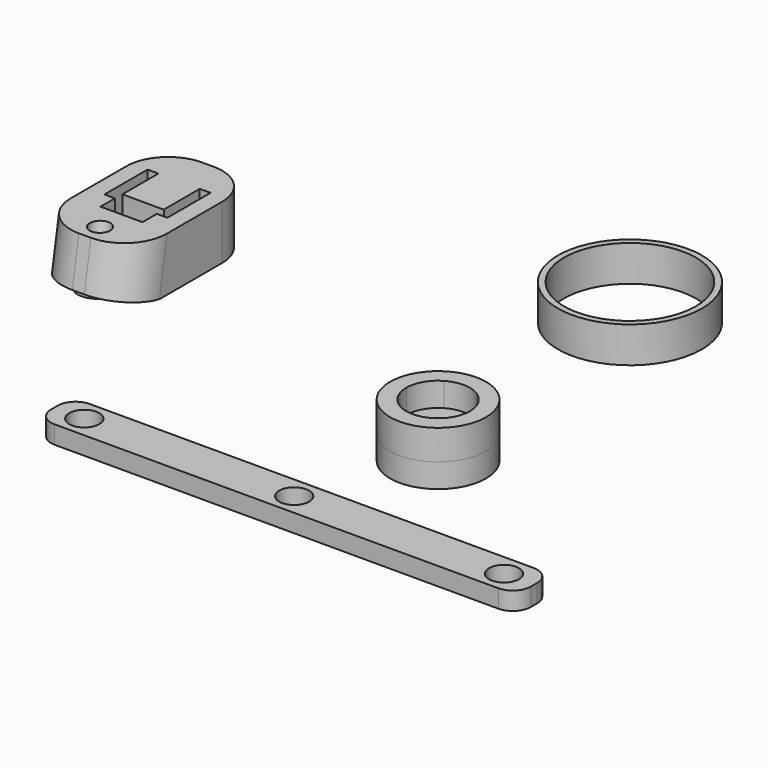
from build123d import *

# Parameters (mm, degrees)
F0_R         = 8
F1_DEPTH     = 4
F2_DEPTH     = 5
F0_R_2       = 2.5
F3_DEPTH     = 1
F4_DEPTH     = 3
F0_R_3       = 12
F0_R_4       = 11
F5_DEPTH     = 6
F0_W         = 16
F0_H         = 7
F0_H_2       = 20
F6_DEPTH     = 9
F8_W         = 16
F8_H         = 7.1079862832
F8_R         = 2.4
F8_R_2       = 1.7
F9_DEPTH     = 11.0033706387
F10_DEPTH    = 16.6784377721
F11_DEPTH    = 0.7
F12_R        = 2.3
F13_DEPTH    = 20
F8_H_2       = 1.3485015869
F14_DEPTH    = 16.6784377721
F15_T1_DEPTH = 44
F15_T3_DEPTH = 42.8855097467


# Not quite as in the source:
# - a fillet or chamfer that OpenCascade refuses, or shapes differently, is made with other operations: its cross-section is extruded or revolved along the edge and cut away or added


with BuildPart() as f1:
    # F0 (on Top) → F1 (new body)
    with BuildSketch(Plane.XY):
        Circle(F0_R)
        Polygon((5.3, 3.0599564267), (5.3, 0), (5.3, -3.0599564267), (2.6500008794, -4.5899341324), (0, -6.1199128534), (-2.6500009439, -4.5899340951), (-5.3, -3.0599564267), (-5.3, 0), (-5.3, 3.0599564267), (-2.6500008588, 4.5899341442), (0, 6.1199128534), (2.6500008831, 4.5899341302), align=None, mode=Mode.SUBTRACT)
    extrude(amount=-F1_DEPTH)

    # F0 (on Top) → F2 (join)
    with BuildSketch(Plane.XY):
        Circle(F0_R)
        Polygon((5.3, 3.0599564267), (5.3, 0), (5.3, -3.0599564267), (2.6500008794, -4.5899341324), (0, -6.1199128534), (-2.6500009439, -4.5899340951), (-5.3, -3.0599564267), (-5.3, 0), (-5.3, 3.0599564267), (-2.6500008588, 4.5899341442), (0, 6.1199128534), (2.6500008831, 4.5899341302), align=None, mode=Mode.SUBTRACT)
        with BuildLine():
            Line((0, -6.1199128534), (2.6500008794, -4.5899341324))
            ThreePointArc((2.6500008794, -4.5899341324), (-3.73e-08, -5.3), (-2.6500009439, -4.5899340951))
            Line((-2.6500009439, -4.5899340951), (0, -6.1199128534))
        make_face()
        with BuildLine():
            Line((-5.3, -3.0599564267), (-2.6500009439, -4.5899340951))
            ThreePointArc((-2.6500009439, -4.5899340951), (-4.5899349125, -2.6499995281), (-5.3, 0))
            Line((-5.3, 0), (-5.3, -3.0599564267))
        make_face()
        with BuildLine():
            ThreePointArc((-5.3, 0), (-4.589934888, 2.6499995706), (-2.6500008588, 4.5899341442))
            Line((-2.6500008588, 4.5899341442), (-5.3, 3.0599564267))
            Line((-5.3, 3.0599564267), (-5.3, 0))
        make_face()
        with BuildLine():
            Line((5.3, -3.0599564267), (5.3, 0))
            ThreePointArc((5.3, 0), (4.5899348939, -2.6499995603), (2.6500008794, -4.5899341324))
            Line((2.6500008794, -4.5899341324), (5.3, -3.0599564267))
        make_face()
        with BuildLine():
            ThreePointArc((2.6500008831, 4.5899341302), (4.589934895, 2.6499995585), (5.3, 0))
            Line((5.3, 0), (5.3, 3.0599564267))
            Line((5.3, 3.0599564267), (2.6500008831, 4.5899341302))
        make_face()
        with BuildLine():
            ThreePointArc((-2.6500008588, 4.5899341442), (1.4e-08, 5.3), (2.6500008831, 4.5899341302))
            Line((2.6500008831, 4.5899341302), (0, 6.1199128534))
            Line((0, 6.1199128534), (-2.6500008588, 4.5899341442))
        make_face()
    extrude(amount=F2_DEPTH)

    # F0 (on Top) → F3 (join)
    with BuildSketch(Plane.XY):
        with BuildLine():
            ThreePointArc((2.6500008794, -4.5899341324), (4.5899348939, -2.6499995603), (5.3, 0))
            ThreePointArc((5.3, 0), (4.589934895, 2.6499995585), (2.6500008831, 4.5899341302))
            ThreePointArc((2.6500008831, 4.5899341302), (1.4e-08, 5.3), (-2.6500008588, 4.5899341442))
            ThreePointArc((-2.6500008588, 4.5899341442), (-4.589934888, 2.6499995706), (-5.3, 0))
            ThreePointArc((-5.3, 0), (-4.5899349125, -2.6499995281), (-2.6500009439, -4.5899340951))
            ThreePointArc((-2.6500009439, -4.5899340951), (-3.73e-08, -5.3), (2.6500008794, -4.5899341324))
        make_face()
        Circle(F0_R_2, mode=Mode.SUBTRACT)
    extrude(amount=F3_DEPTH)


with BuildPart() as f4:
    # F0 (on Top) → F4 (new body)
    with BuildSketch(Plane.XY):
        with BuildLine():
            Line((-37, -33.675), (37, -33.675))
            ThreePointArc((37, -33.675), (39.1213203436, -32.7963203436), (40, -30.675))
            Line((40, -30.675), (40, -29.325))
            ThreePointArc((40, -29.325), (39.1213203436, -27.2036796564), (37, -26.325))
            Line((37, -26.325), (-37, -26.325))
            ThreePointArc((-37, -26.325), (-39.1213203436, -27.2036796564), (-40, -29.325))
            Line((-40, -29.325), (-40, -30.675))
            ThreePointArc((-40, -30.675), (-39.1213203436, -32.7963203436), (-37, -33.675))
        make_face()
        with Locations((-35, -30)):
            Circle(F0_R_2, mode=Mode.SUBTRACT)
        with Locations((0, -30)):
            Circle(F0_R_2, mode=Mode.SUBTRACT)
        with Locations((35, -30)):
            Circle(F0_R_2, mode=Mode.SUBTRACT)
    extrude(amount=F4_DEPTH)


with BuildPart() as f5:
    # F0 (on Top) → F5 (new body)
    with BuildSketch(Plane.XY):
        with Locations((0, 40)):
            Circle(F0_R_3)
        with Locations((0, 40)):
            Circle(F0_R_4, mode=Mode.SUBTRACT)
    extrude(amount=F5_DEPTH)


with BuildPart() as f6:
    # F0 (on Top) → F6 (new body)
    with BuildSketch(Plane.XY):
        with Locations((-60, 3.5)):
            Rectangle(F0_W, F0_H)
        with Locations((-60, 17)):
            Rectangle(F0_W, F0_H_2)
        Polygon((-65.25, 12), (-65.25, 21), (-63.45, 21), (-63.45, 13.5), (-56.55, 13.5), (-56.55, 21), (-54.75, 21), (-54.75, 12), (-56.5, 12), (-56.5, 9), (-63.5, 9), (-63.5, 12), align=None, mode=Mode.SUBTRACT)
    extrude(amount=F6_DEPTH)

    # F8 (on line) → F9 (cut, through all)
    with BuildSketch(Plane(origin=(0, 0.2110758272, 1.1970705016), x_dir=(1, 0, 0), z_dir=(0, -0.1736481777, -0.984807753))):
        with Locations((-60, -3.3396611295)):
            Rectangle(F8_W, F8_H)
        with Locations((-60, -2.8936542711)):
            Circle(F8_R, mode=Mode.SUBTRACT)
        with Locations((-60, -2.8936542711)):
            Circle(F8_R)
        with Locations((-60, -2.8936542711)):
            Circle(F8_R_2, mode=Mode.SUBTRACT)
        with Locations((-60, -2.8936542711)):
            Circle(F8_R_2)
    extrude(amount=F9_DEPTH, mode=Mode.SUBTRACT)

    # F8 (on line) → F10 (cut, through all)
    with BuildSketch(Plane(origin=(0, 0.2110758272, 1.1970705016), x_dir=(1, 0, 0), z_dir=(0, -0.1736481777, -0.984807753))):
        with Locations((-60, -2.8936542711)):
            Circle(F8_R_2)
    extrude(amount=-F10_DEPTH, mode=Mode.SUBTRACT)

    # F8 (on line) → F11 (join)
    with BuildSketch(Plane(origin=(0, 0.2110758272, 1.1970705016), x_dir=(1, 0, 0), z_dir=(0, -0.1736481777, -0.984807753))):
        with Locations((-60, -2.8936542711)):
            Circle(F8_R)
        with Locations((-60, -2.8936542711)):
            Circle(F8_R_2, mode=Mode.SUBTRACT)
    extrude(amount=F11_DEPTH)

    # F12 (on face) → F13 (cut)
    with BuildSketch(Plane(origin=(0, 27, 0), x_dir=(-1, 0, 0), z_dir=(0, 1, 0))):
        with Locations((60, 3.1)):
            Circle(F12_R)
    extrude(amount=-F13_DEPTH, mode=Mode.SUBTRACT)

    # F8 (on line) → F14 (cut, through all)
    with BuildSketch(Plane(origin=(0, 0.2110758272, 1.1970705016), x_dir=(1, 0, 0), z_dir=(0, -0.1736481777, -0.984807753))):
        with Locations((-60, 0.8885828056)):
            Rectangle(F8_W, F8_H_2)
    extrude(amount=-F14_DEPTH, mode=Mode.SUBTRACT)

    # F15: fillet of radius 7 on 4 edges, made by hand

    # F15_s2 → F15_t1 (cut)
    with BuildSketch(Plane.XY.offset(-17.5)):
        with BuildLine():
            ThreePointArc((-52, 20), (-54.0502525317, 24.9497474683), (-59, 27))
            Line((-59, 27), (-52, 27))
            Line((-52, 27), (-52, 20))
        make_face()
        with BuildLine():
            ThreePointArc((-68, 20), (-65.9497474683, 24.9497474683), (-61, 27))
            Line((-61, 27), (-68, 27))
            Line((-68, 27), (-68, 20))
        make_face()
    extrude(amount=F15_T1_DEPTH, mode=Mode.SUBTRACT)

    # F15_s4 → F15_t3 (cut)
    with BuildSketch(Plane(origin=(0, -2.8277672819, -16.0370651761), x_dir=(1, 0, 0), z_dir=(0, 0.1736481777, 0.984807753))):
        with BuildLine():
            ThreePointArc((-52, 6.7856679879), (-54.0502525317, 1.8359205196), (-59, -0.2143320121))
            Line((-59, -0.2143320121), (-52, -0.2143320121))
            Line((-52, -0.2143320121), (-52, 6.7856679879))
        make_face()
        with BuildLine():
            ThreePointArc((-68, 6.7856679879), (-65.9497474683, 1.8359205196), (-61, -0.2143320121))
            Line((-61, -0.2143320121), (-68, -0.2143320121))
            Line((-68, -0.2143320121), (-68, 6.7856679879))
        make_face()
    extrude(amount=F15_T3_DEPTH, mode=Mode.SUBTRACT)


solid = Compound([f1.part, f4.part, f5.part, f6.part])
